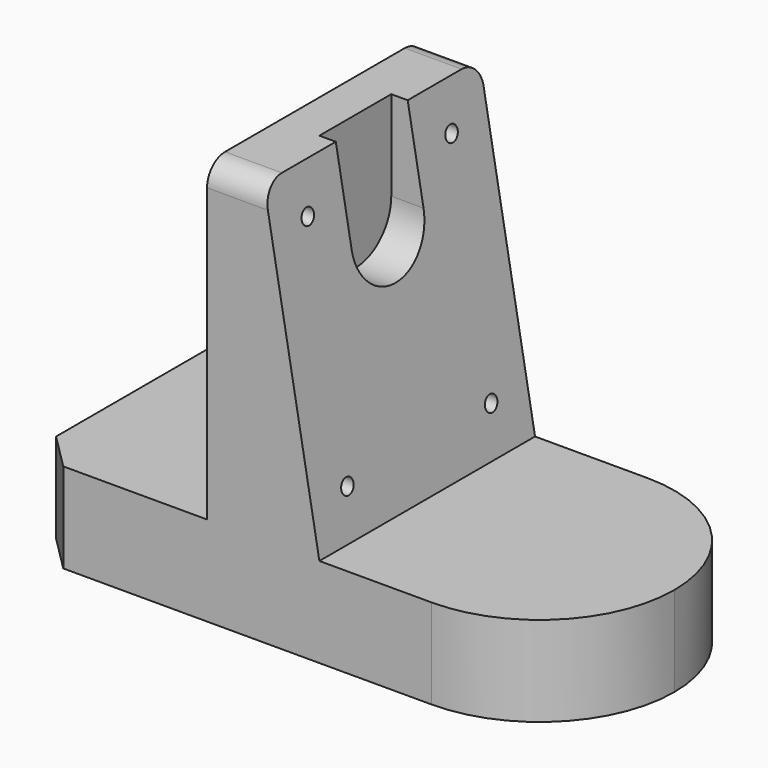
from build123d import *

# Parameters (mm, degrees)
F1_DEPTH       = 30
F2_R           = 29.99999
F4_D           = 3.4
F4_CBORE_D     = 7
F4_CBORE_DEPTH = 2
F5_SIZE        = 8
F10_DEPTH      = 16
F11_DEPTH      = 60.001
F12_R          = 5


# Not quite as in the source:
# - a fillet or chamfer is up to 0.001 mm smaller than in the source, because OpenCascade refuses the exact size


with BuildPart() as f1:
    # F0 (on Front) → F1 (new body, symmetric)
    with BuildSketch(Plane.XZ):
        Polygon((0, 20), (0, 0), (120, 0), (120, 20), (65, 20), (65, 90), (40, 90), (40, 20), align=None)
    extrude(amount=F1_DEPTH, both=True)

    # F2 (radius 30 in the source; OpenCascade refuses exactly that, so slightly less here)
    f2_edges = [f1.edges().sort_by_distance(p)[0] for p in [
        (120, -30, 10),
        (120, 30, 10),
    ]]
    fillet(f2_edges, radius=F2_R)

    # F4 (through all)
    with Locations(Plane(origin=(40, 0, 0), x_dir=(0, -1, 0), z_dir=(-1, 0, 0))):
        with Locations((-20, 80), (-20, 30), (20, 30), (20, 80)):
            CounterBoreHole(F4_D / 2, F4_CBORE_D / 2, F4_CBORE_DEPTH)

    # F5
    f5_edges = [f1.edges().sort_by_distance(p)[0] for p in [
        (0, 30, 10),
        (0, -30, 10),
    ]]
    chamfer(f5_edges, length=F5_SIZE)

    # F7 (on face) → F10 (cut, through all)
    with BuildSketch(Plane.YZ.offset(65)):
        with BuildLine():
            ThreePointArc((-10, 70), (0, 80), (10, 70))
            Line((10, 70), (10, 90))
            Line((10, 90), (-10, 90))
            Line((-10, 90), (-10, 70))
        make_face()
        with BuildLine():
            ThreePointArc((-10, 70), (0, 60), (10, 70))
            ThreePointArc((10, 70), (0, 80), (-10, 70))
        make_face()
    extrude(amount=-F10_DEPTH, mode=Mode.SUBTRACT)

    # F6 (on face) → F11 (cut, through all)
    with BuildSketch(Plane.XZ.offset(30)):
        Polygon((52.6571113504, 90), (65, 20), (65, 90), align=None)
    extrude(amount=-F11_DEPTH, mode=Mode.SUBTRACT)

    # F12
    f12_edges = [f1.edges().sort_by_distance(p)[0] for p in [
        (46.328556, -30, 90),
        (46.328556, 30, 90),
    ]]
    fillet(f12_edges, radius=F12_R)


solid = f1.part
